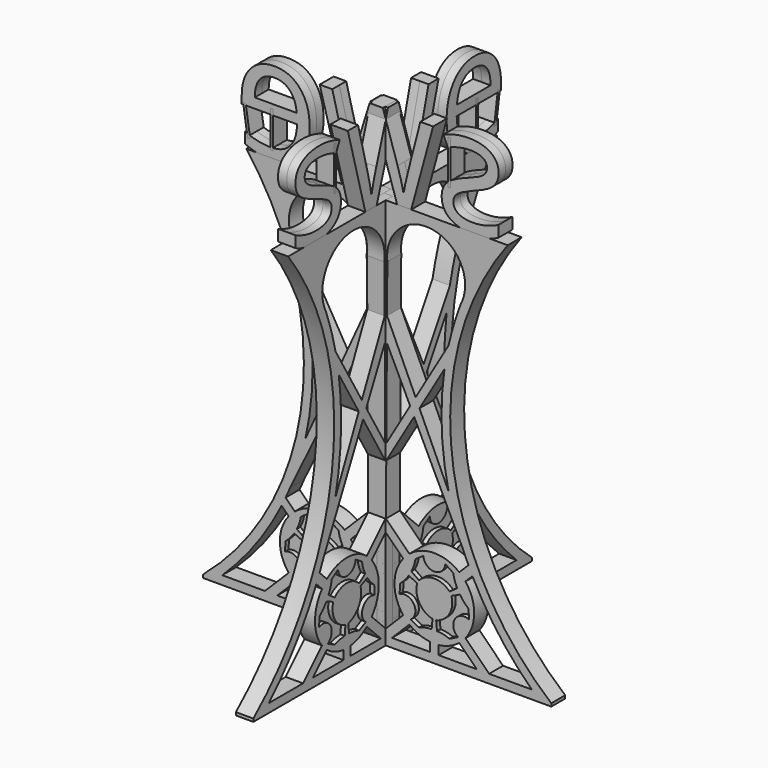
from build123d import *

# Parameters (mm, degrees)
F1_DEPTH       = 2
F1_DEPTH_BACK  = 2
F3_COUNT       = 4
F3_ANGLE       = 270
F4_TEXT_SIZE   = 34.4529419737
F5_DEPTH       = 2
F5_DEPTH_BACK  = 2
F7_W           = 0.6
F7_H           = 10.0924548263
F8_DEPTH       = 2
F8_DEPTH_BACK  = 2
F7_H_2         = 8.4090257245
F9_COUNT       = 2
F9_ANGLE       = 90
F10_R          = 8.718741745
F12_DEPTH      = 1
F12_DEPTH_BACK = 1
F13_COUNT      = 4
F13_ANGLE      = 270


# Not quite as in the source:
# - Text() gives the source's letters only with a copy of the font that has no kerning and outlines rounded to 1/6400 em; it was checked with that copy


with BuildPart() as f1:
    # F0 (on Right) → F1 (new body, two sides)
    with BuildSketch(Plane.YZ) as f1_sk:
        with BuildLine():
            Line((0, 90), (-30, 90))
            ThreePointArc((-30, 90), (-17.2003120889, 43.34622274), (-40, 0.6779537991))
            Line((-40, 0.6779537991), (-40, 0))
            Line((-40, 0), (0, 0))
            Line((0, 0), (0, 90))
        make_face()
        with BuildLine():
            Line((-25.7327414086, 2), (-35.5405993869, 2))
            ThreePointArc((-35.5405993869, 2), (-27.9283935316, 10.6626442463), (-21.9059731011, 20.4971516301))
            Line((-21.9059731011, 20.4971516301), (-20.2955077074, 18.8856066293))
            ThreePointArc((-20.2955077074, 18.8856066293), (-22.3105750639, 13.1583554739), (-20.2993462482, 7.4297552174))
            Line((-20.2993462482, 7.4297552174), (-25.7327414086, 2))
        make_face(mode=Mode.SUBTRACT)
        with BuildLine():
            Line((-14.1552877889, 2), (-22.9033660792, 2))
            Line((-22.9033660792, 2), (-18.8856066293, 6.0150678704))
            ThreePointArc((-18.8856066293, 6.0150678704), (-16.6602817808, 4.6974918813), (-14.1552877889, 4.0547771165))
            Line((-14.1552877889, 4.0547771165), (-14.1552877889, 2))
        make_face(mode=Mode.SUBTRACT)
        with BuildLine():
            Line((-16.6618152555, 6.1222817374), (-18.6122404521, 7.0947278683))
            ThreePointArc((-18.6122404521, 7.0947278683), (-17.8389383596, 10.4511808711), (-21.1323629729, 11.4597081156))
            Line((-21.1323629729, 11.4597081156), (-20.9993134278, 13.6350489495))
            ThreePointArc((-20.9993134278, 13.6350489495), (-19.9158795248, 14.6446345056), (-19.0341370726, 15.8344337598))
            Line((-19.0341370726, 15.8344337598), (-17.0775409464, 14.9427615336))
            ThreePointArc((-17.0775409464, 14.9427615336), (-16.6204800926, 11.1546580796), (-13.5684166961, 8.864780042))
            Line((-13.5684166961, 8.864780042), (-13.7745039595, 6.7244819787))
            ThreePointArc((-13.7745039595, 6.7244819787), (-15.2457715651, 6.5557702426), (-16.6618152555, 6.1222817374))
        make_face(mode=Mode.SUBTRACT)
        with BuildLine():
            Line((-7.8956546758, 16.9069476282), (-9.6461635386, 15.658321791))
            ThreePointArc((-9.6461635386, 15.658321791), (-13.1552877889, 17.1565472076), (-16.6644120392, 15.658321791))
            Line((-16.6644120392, 15.658321791), (-18.414920902, 16.9069476282))
            ThreePointArc((-18.414920902, 16.9069476282), (-17.8253957486, 18.2654586185), (-17.4927859612, 19.7085326798))
            Line((-17.4927859612, 19.7085326798), (-15.6754103097, 20.9114273828))
            ThreePointArc((-15.6754103097, 20.9114273828), (-13.1552877889, 18.5635016245), (-10.6351652681, 20.9114273828))
            Line((-10.6351652681, 20.9114273828), (-8.8177896166, 19.7085326798))
            ThreePointArc((-8.8177896166, 19.7085326798), (-8.4851798292, 18.2654586185), (-7.8956546758, 16.9069476282))
        make_face(mode=Mode.SUBTRACT)
        with BuildLine():
            Line((-7.4297552174, 6.0112293296), (-3.4212130927, 2))
            Line((-3.4212130927, 2), (-12.1552877889, 2))
            Line((-12.1552877889, 2), (-12.1552877889, 4.0547771165))
            ThreePointArc((-12.1552877889, 4.0547771165), (-9.6531279684, 4.6963179291), (-7.4297552174, 6.0112293296))
        make_face(mode=Mode.SUBTRACT)
        with BuildLine():
            Line((-5.31126215, 13.6350489495), (-5.1782126049, 11.4597081156))
            ThreePointArc((-5.1782126049, 11.4597081156), (-8.4716372182, 10.4511808711), (-7.6983351257, 7.0947278683))
            Line((-7.6983351257, 7.0947278683), (-9.6487603223, 6.1222817374))
            ThreePointArc((-9.6487603223, 6.1222817374), (-11.0648040127, 6.5557702426), (-12.5360716183, 6.7244819787))
            Line((-12.5360716183, 6.7244819787), (-12.7421588817, 8.864780042))
            ThreePointArc((-12.7421588817, 8.864780042), (-9.6900954852, 11.1546580796), (-9.2330346314, 14.9427615336))
            Line((-9.2330346314, 14.9427615336), (-7.2764385052, 15.8344337598))
            ThreePointArc((-7.2764385052, 15.8344337598), (-6.394696053, 14.6446345056), (-5.31126215, 13.6350489495))
        make_face(mode=Mode.SUBTRACT)
        with BuildLine():
            Line((-1.999999989, 3.4072094877), (-6.0150678704, 7.4249689485))
            ThreePointArc((-6.0150678704, 7.4249689485), (-4.0000005139, 13.1522201039), (-6.0112293296, 18.8808203604))
            Line((-6.0112293296, 18.8808203604), (-2, 22.8893624851))
            Line((-2, 22.8893624851), (-2, 3.4072094877))
        make_face(mode=Mode.SUBTRACT)
        with BuildLine():
            Line((-18.8808203604, 20.2993462482), (-20.9877872685, 22.4077256029))
            ThreePointArc((-20.9877872685, 22.4077256029), (-20.4565558144, 23.5889353751), (-19.9481418942, 24.7801442859))
            Line((-19.9481418942, 24.7801442859), (-8.5133343285, 48.3528648343))
            Line((-8.5133343285, 48.3528648343), (-2.1230393044, 37.4420163971))
            Line((-2.1230393044, 37.4420163971), (-2.0520642774, 25.6648129594))
            Line((-2.0520642774, 25.6648129594), (-7.4249689485, 20.2955077074))
            ThreePointArc((-7.4249689485, 20.2955077074), (-13.1522201039, 22.3105750639), (-18.8808203604, 20.2993462482))
        make_face(mode=Mode.SUBTRACT)
        with BuildLine():
            Line((-9.7440407185, 50.454184232), (-16.4474927484, 35.7879071738))
            ThreePointArc((-16.4474927484, 35.7879071738), (-14.846182039, 47.982119379), (-15.4895860027, 60.2641810395))
            Line((-15.4895860027, 60.2641810395), (-9.7440407185, 50.454184232))
        make_face(mode=Mode.SUBTRACT)
        Polygon((-7.5962813104, 50.2433587846), (-2.2664020758, 61.2308417863), (-2.1440850364, 40.9342287726), align=None, mode=Mode.SUBTRACT)
        with BuildLine():
            ThreePointArc((-19.1737074097, 74.5014338268), (-12.932358817, 87.5294981022), (-2.3655281282, 77.6792706828))
            Line((-2.3655281282, 77.6792706828), (-2.2996126455, 66.7416200443))
            Line((-2.2996126455, 66.7416200443), (-8.8567412124, 52.3954796022))
            Line((-8.8567412124, 52.3954796022), (-16.4158863474, 65.302033458))
            ThreePointArc((-16.4158863474, 65.302033458), (-17.6305752624, 69.9509644415), (-19.1737074097, 74.5014338268))
        make_face(mode=Mode.SUBTRACT)
    extrude(amount=F1_DEPTH)
    extrude(f1_sk.sketch, amount=-F1_DEPTH_BACK)


with BuildPart() as f3_1:
    # F3: instance of F1
    add(f1.part.rotate(Axis((0, 0, 26.2590656057), (0, 0, -1)), 1 * F3_ANGLE / (F3_COUNT - 1)))


with BuildPart() as f3_2:
    # F3: instance of F1
    add(f1.part.rotate(Axis((0, 0, 26.2590656057), (0, 0, -1)), 2 * F3_ANGLE / (F3_COUNT - 1)))

    # F10 (on Right) → F12 (join, two sides)
    with BuildSketch(Plane.YZ) as f12_sk:
        with Locations((13.1552877889, 13.1552877889)):
            Circle(F10_R)
    extrude(amount=F12_DEPTH)
    extrude(f12_sk.sketch, amount=-F12_DEPTH_BACK)


with BuildPart() as f3_3:
    # F3: instance of F1
    add(f1.part.rotate(Axis((0, 0, 26.2590656057), (0, 0, -1)), 3 * F3_ANGLE / (F3_COUNT - 1)))


with BuildPart() as f5:
    # F4 (on Right) → F5 (new body, two sides)
    with BuildSketch(Plane.YZ) as f5_sk:
        with Locations((-29.6972369404, 90)):
            Text('swe', F4_TEXT_SIZE, font='Open Sans', text_align=(TextAlign.LEFT, TextAlign.BOTTOM))
    extrude(amount=F5_DEPTH)
    extrude(f5_sk.sketch, amount=-F5_DEPTH_BACK)


with BuildPart() as f8:
    # F7 (on Right) → F8 (new body, two sides)
    with BuildSketch(Plane.YZ) as f8_sk:
        with Locations((-16.6137714344, 102.3634375158)):
            Rectangle(F7_W, F7_H)
    extrude(amount=F8_DEPTH)
    extrude(f8_sk.sketch, amount=-F8_DEPTH_BACK)


with BuildPart() as f8b:
    # F7 (on Right) → F8, piece 2 (new body, two sides)
    with BuildSketch(Plane.YZ) as f8_2_sk:
        Polygon((30.75383332, 99.1032102112), (30.15383332, 99.1032102112), (29.1138019592, 92.2848388378), (29.7138019592, 92.2848388378), align=None)
    extrude(amount=F8_DEPTH)
    extrude(f8_2_sk.sketch, amount=-F8_DEPTH_BACK)


with BuildPart() as f8c:
    # F7 (on Right) → F8, piece 3 (new body, two sides)
    with BuildSketch(Plane.YZ) as f8_3_sk:
        with Locations((24.1984159872, 95.7529542723)):
            Rectangle(F7_W, F7_H_2)
    extrude(amount=F8_DEPTH)
    extrude(f8_3_sk.sketch, amount=-F8_DEPTH_BACK)


with BuildPart() as f9_1:
    # F9: instance of F5
    add(f5.part.rotate(Axis((0, 0, 82.2183042765), (0, 0, 1)), 1 * F9_ANGLE / (F9_COUNT - 1)))


with BuildPart() as f9_2:
    # F9: instance of F8
    add(f8.part.rotate(Axis((0, 0, 82.2183042765), (0, 0, 1)), 1 * F9_ANGLE / (F9_COUNT - 1)))


with BuildPart() as f9_3:
    # F9: instance of F8b
    add(f8b.part.rotate(Axis((0, 0, 82.2183042765), (0, 0, 1)), 1 * F9_ANGLE / (F9_COUNT - 1)))


with BuildPart() as f9_4:
    # F9: instance of F8c
    add(f8c.part.rotate(Axis((0, 0, 82.2183042765), (0, 0, 1)), 1 * F9_ANGLE / (F9_COUNT - 1)))


with BuildPart() as f13_1:
    # F13: instance of F3_2
    add(f3_2.part.rotate(Axis((0, 0, -9.0715694241), (0, 0, -1)), 1 * F13_ANGLE / (F13_COUNT - 1)))


with BuildPart() as f13_2:
    # F13: instance of F3_2
    add(f3_2.part.rotate(Axis((0, 0, -9.0715694241), (0, 0, -1)), 2 * F13_ANGLE / (F13_COUNT - 1)))


with BuildPart() as f13_3:
    # F13: instance of F3_2
    add(f3_2.part.rotate(Axis((0, 0, -9.0715694241), (0, 0, -1)), 3 * F13_ANGLE / (F13_COUNT - 1)))


solid = Compound([f1.part, f3_1.part, f3_2.part, f3_3.part, f5.part, f8.part, f8b.part, f8c.part, f9_1.part, f9_2.part, f9_3.part, f9_4.part, f13_1.part, f13_2.part, f13_3.part])
